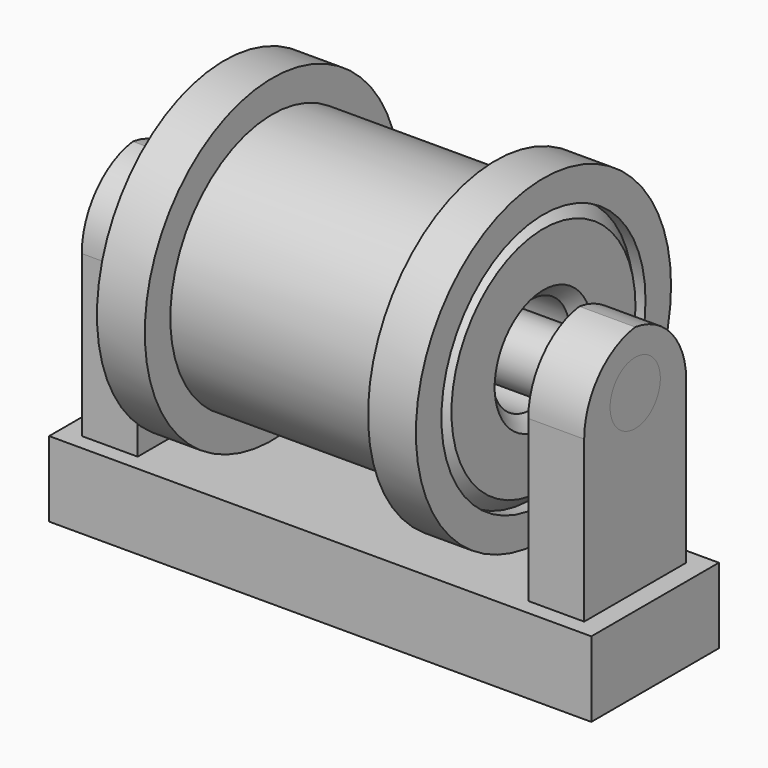
from build123d import *

# Parameters (mm, degrees)
F0_W          = 43.18
F0_H          = 12.7
F0_W_2        = 4.4527295977
F0_H_2        = 10.16
F0_W_3        = 4.4527407736
F1_DEPTH      = 6
F2_START      = 0.19698
F2_DEPTH      = 24.44102
F3_T1_DEPTH   = 33.6627407736
F3_2_T1_DEPTH = 33.6627295977
F4_R          = 2.5
F5_DEPTH      = 40.0127351856
F6_DEPTH      = 40.0127351856
F7_R          = 12.7
F7_R_2        = 10.16
F8_DEPTH      = 12.7
F7_R_3        = 3.8600941061
F9_DEPTH      = 12.7
F10_DEPTH     = 8.89
F11_SIZE      = 1


# Not quite as in the source:
# - a fillet or chamfer that OpenCascade refuses, or shapes differently, is made with other operations: its cross-section is extruded or revolved along the edge and cut away or added


with BuildPart() as f1:
    # F0 (on Top) → F1 (new body)
    with BuildSketch(Plane.XY):
        Rectangle(F0_W, F0_H)
        with Locations((-17.78, 0)):
            Rectangle(F0_W_2, F0_H_2, mode=Mode.SUBTRACT)
        with Locations((17.78, 0)):
            Rectangle(F0_W_3, F0_H_2, mode=Mode.SUBTRACT)
    extrude(amount=F1_DEPTH)


with BuildPart() as f2:
    # F0 (on Top) → F2 (new body)
    with BuildSketch(Plane.XY.offset(F2_START)):
        with Locations((-17.78, 0)):
            Rectangle(F0_W_2, F0_H_2)
    extrude(amount=F2_DEPTH)

    # F3#2: fillet of radius 5.842 on 2 edges, made by hand

    # F3_2_s2 → F3_2_t1 (cut)
    with BuildSketch(Plane.YZ.offset(-34.6113647988)):
        with BuildLine():
            ThreePointArc((5.08, 18.796), (3.3689178157, 22.9269178157), (-0.762, 24.638))
            Line((-0.762, 24.638), (5.08, 24.638))
            Line((5.08, 24.638), (5.08, 18.796))
        make_face()
        with BuildLine():
            ThreePointArc((-5.08, 18.796), (-3.3689178157, 22.9269178157), (0.762, 24.638))
            Line((0.762, 24.638), (-5.08, 24.638))
            Line((-5.08, 24.638), (-5.08, 18.796))
        make_face()
    extrude(amount=F3_2_T1_DEPTH, mode=Mode.SUBTRACT)


with BuildPart() as f2b:
    # F0 (on Top) → F2, piece 2 (new body)
    with BuildSketch(Plane.XY.offset(F2_START)):
        with Locations((17.78, 0)):
            Rectangle(F0_W_3, F0_H_2)
    extrude(amount=F2_DEPTH)

    # F3: fillet of radius 5.842 on 2 edges, made by hand

    # F3_s2 → F3_t1 (cut)
    with BuildSketch(Plane.YZ.offset(0.9486296132)):
        with BuildLine():
            ThreePointArc((5.08, 18.796), (3.3689178157, 22.9269178157), (-0.762, 24.638))
            Line((-0.762, 24.638), (5.08, 24.638))
            Line((5.08, 24.638), (5.08, 18.796))
        make_face()
        with BuildLine():
            ThreePointArc((-5.08, 18.796), (-3.3689178157, 22.9269178157), (0.762, 24.638))
            Line((0.762, 24.638), (-5.08, 24.638))
            Line((-5.08, 24.638), (-5.08, 18.796))
        make_face()
    extrude(amount=F3_T1_DEPTH, mode=Mode.SUBTRACT)


with BuildPart() as f5_tool:
    # F4 (on face) → F5 (new body, through all)
    with BuildSketch(Plane(origin=(-20.0063647988, 0, 0), x_dir=(0, -1, 0), z_dir=(-1, 0, 0))):
        with Locations((0, 19.97)):
            Circle(F4_R)
    extrude(amount=-F5_DEPTH)


with BuildPart() as f2_1:
    add(f2.part)

    # F5: cut by f5_tool
    add(f5_tool.part, mode=Mode.SUBTRACT)


with BuildPart() as f2b_1:
    add(f2b.part)

    # F5: cut by f5_tool
    add(f5_tool.part, mode=Mode.SUBTRACT)


with BuildPart() as f6:
    # F4 (on face) → F6 (new body, through all)
    with BuildSketch(Plane(origin=(-20.0063647988, 0, 0), x_dir=(0, -1, 0), z_dir=(-1, 0, 0))):
        with Locations((0, 19.97)):
            Circle(F4_R)
    extrude(amount=-F6_DEPTH)


with BuildPart() as f8:
    # F7 (on Right) → F8 (new body, symmetric)
    with BuildSketch(Plane.YZ):
        with Locations((0, 19.9550520629)):
            Circle(F7_R)
        with Locations((0, 19.9550520629)):
            Circle(F7_R_2, mode=Mode.SUBTRACT)
    extrude(amount=F8_DEPTH, both=True)

    # F7 (on Right) → F10 (cut, symmetric)
    with BuildSketch(Plane.YZ):
        with Locations((0, 19.9550520629)):
            Circle(F7_R)
        with Locations((0, 19.9550520629)):
            Circle(F7_R_2, mode=Mode.SUBTRACT)
    extrude(amount=F10_DEPTH, both=True, mode=Mode.SUBTRACT)


with BuildPart() as f9:
    # F7 (on Right) → F9 (new body, symmetric)
    with BuildSketch(Plane.YZ):
        with Locations((0, 19.9550520629)):
            Circle(F7_R_2)
        with Locations((0, 19.9550520629)):
            Circle(F7_R_3, mode=Mode.SUBTRACT)
    extrude(amount=F9_DEPTH, both=True)

    # F11
    f11_edges = [f9.edges().sort_by_distance(p)[0] for p in [
        (12.7, -3.860094, 19.955052),
        (-12.7, -3.860094, 19.955052),
        (12.7, -10.16, 19.955052),
        (-12.7, -10.16, 19.955052),
        (0, 10.16, 19.955052),
    ]]
    chamfer(f11_edges, length=F11_SIZE)


solid = Compound([f1.part, f2_1.part, f2b_1.part, f6.part, f8.part, f9.part])
